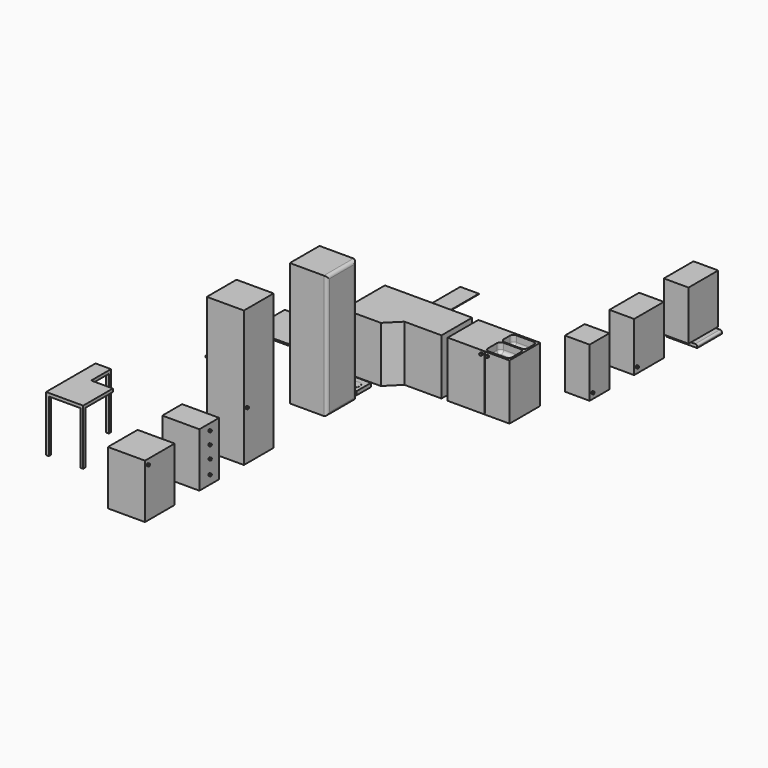
from build123d import *

# Parameters (mm, degrees)
F1_W           = 600
F1_H           = 600
F2_DEPTH       = 2000
F1_W_2         = 520
F1_H_2         = 290
F1_R           = 100
F1_R_2         = 80
F3_DEPTH       = 60
F4_DEPTH       = 900
F1_W_3         = 1000
F1_H_3         = 620
F5_DEPTH       = 900
F7_DEPTH       = 150
F8_R           = 50
F9_T           = 15
F10_DEPTH      = 61
F1_H_4         = 400
F11_DEPTH      = 875
F1_W_4         = 400
F1_H_5         = 50
F1_H_6         = 500
F12_DEPTH      = 800
F1_W_5         = 100
F13_DEPTH      = 50
F14_R          = 30
F15_DEPTH      = 800
F1_W_6         = 620
F1_H_7         = 700
F16_DEPTH      = 25
F17_R          = 20
F18_DEPTH      = 25
F19_DEPTH      = 2200
F20_R          = 20
F21_DEPTH      = 25
F22_R          = 50
F23_W          = 584
F23_H          = 870
F23_R          = 20
F23_W_2        = 385
F24_DEPTH      = 12
F25_DEPTH      = 25
F25_DEPTH_BACK = 12
F1_W_7         = 300
F1_H_8         = 900
F26_DEPTH      = 9
F1_W_8         = 45
F1_H_9         = 45
F27_DEPTH      = 50
F28_DEPTH      = 900


# Not quite as in the source:
# - a shell that OpenCascade refuses in one call is made with other operations: the cavity is built on its own and cut out


with BuildPart() as f2:
    # F1 (on Top) → F2 (new body)
    with BuildSketch(Plane.XY):
        with Locations((301, -1623.132034356)):
            Rectangle(F1_W, F1_H)
    extrude(amount=F2_DEPTH)

    # F22
    f22_edges = [f2.edges().sort_by_distance(p)[0] for p in [
        (601, -1923.132034, 1000),
        (601, -1323.132034, 1000),
        (601, -1623.132034, 2000),
        (601, -1623.132034, 0),
    ]]
    fillet(f22_edges, radius=F22_R)


with BuildPart() as f3:
    # F1 (on Top) → F3 (new body)
    with BuildSketch(Plane.XY):
        with Locations((261, -1078.132034356)):
            Rectangle(F1_W_2, F1_H_2)
        with Locations((181, -1073.132034356)):
            Circle(F1_R, mode=Mode.SUBTRACT)
        with Locations((391, -1093.132034356)):
            Circle(F1_R_2, mode=Mode.SUBTRACT)
    extrude(amount=F3_DEPTH)

    # F1 (on Top) → F10 (join)
    with BuildSketch(Plane.XY):
        with Locations((181, -1073.132034356)):
            Circle(F1_R)
        with Locations((391, -1093.132034356)):
            Circle(F1_R_2)
    extrude(amount=F10_DEPTH)


with BuildPart() as f4:
    # F1 (on Top) → F4 (new body)
    with BuildSketch(Plane.XY):
        Polygon((1, -833.132034356), (601, -833.132034356), (813.132034356, -621), (1413.132034356, -621), (1413.132034356, -1), (1, -1), align=None)
    extrude(amount=F4_DEPTH)


with BuildPart() as f5:
    # F1 (on Top) → F5 (new body)
    with BuildSketch(Plane.XY):
        with Locations((2013.132034356, -311)):
            Rectangle(F1_W_3, F1_H_3)
    extrude(amount=F5_DEPTH)

    # F6 (on face) → F7 (cut)
    with BuildSketch(Plane.XY.offset(900)):
        with BuildLine():
            Line((2423.132034356, -291), (2153.132034356, -291))
            ThreePointArc((2153.132034356, -291), (2110.7056274848, -308.5735931288), (2093.132034356, -351))
            Line((2093.132034356, -351), (2093.132034356, -531))
            ThreePointArc((2093.132034356, -531), (2110.7056274848, -573.4264068712), (2153.132034356, -591))
            Line((2153.132034356, -591), (2423.132034356, -591))
            ThreePointArc((2423.132034356, -591), (2465.5584412272, -573.4264068712), (2483.132034356, -531))
            Line((2483.132034356, -531), (2483.132034356, -351))
            ThreePointArc((2483.132034356, -351), (2465.5584412272, -308.5735931288), (2423.132034356, -291))
        make_face()
        with BuildLine():
            ThreePointArc((2093.132034356, -211), (2110.7056274848, -253.4264068712), (2153.132034356, -271))
            Line((2153.132034356, -271), (2423.132034356, -271))
            ThreePointArc((2423.132034356, -271), (2465.5584412272, -253.4264068712), (2483.132034356, -211))
            Line((2483.132034356, -211), (2483.132034356, -91))
            ThreePointArc((2483.132034356, -91), (2465.5584412272, -48.5735931288), (2423.132034356, -31))
            Line((2423.132034356, -31), (2153.132034356, -31))
            ThreePointArc((2153.132034356, -31), (2110.7056274848, -48.5735931288), (2093.132034356, -91))
            Line((2093.132034356, -91), (2093.132034356, -211))
        make_face()
    extrude(amount=-F7_DEPTH, mode=Mode.SUBTRACT)

    # F8
    f8_edges = [f5.edges().sort_by_distance(p)[0] for p in [
        (2288.132034, -291, 750),
        (2288.132034, -31, 750),
    ]]
    fillet(f8_edges, radius=F8_R)

    # F9: shell of thickness 15, made by hand


with BuildPart() as f9_core1:
    # F9_t2: copy of F5
    add(f5.part)

    # the walls: a layer under each face that stays
    f9_faces = [f9_core1.faces().sort_by_distance(p)[0] for p in [
        (2465.5584412272, -308.5735931288, 850),
        (2483.132034356, -441, 850),
        (2455.2031021678, -318.9289321881, 764.6446609407),
        (2013.132034356, -311, 900),
        (2288.132034356, -291, 850),
        (2465.5584412272, -573.4264068712, 850),
        (2468.4873734153, -441, 764.6446609407),
        (2288.132034356, -441, 750),
        (2288.132034356, -305.6446609407, 764.6446609407),
        (1513.132034356, -311, 450),
        (2513.132034356, -311, 450),
        (2013.132034356, -1, 450),
        (2110.7056274848, -308.5735931288, 850),
        (2093.132034356, -441, 850),
        (2110.7056274848, -573.4264068712, 850),
        (2288.132034356, -591, 850),
        (2110.7056274848, -48.5735931288, 850),
        (2093.132034356, -151, 850),
        (2110.7056274848, -253.4264068712, 850),
        (2288.132034356, -271, 850),
        (2465.5584412272, -253.4264068712, 850),
        (2483.132034356, -151, 850),
        (2465.5584412272, -48.5735931288, 850),
        (2288.132034356, -31, 850),
        (2455.2031021678, -563.0710678119, 764.6446609407),
        (2121.0609665441, -318.9289321881, 764.6446609407),
        (2107.7766952966, -441, 764.6446609407),
        (2121.0609665441, -563.0710678119, 764.6446609407),
        (2288.132034356, -576.3553390593, 764.6446609407),
        (2013.132034356, -311, 0),
        (2121.0609665441, -58.9289321881, 764.6446609407),
        (2107.7766952966, -151, 764.6446609407),
        (2121.0609665441, -243.0710678119, 764.6446609407),
        (2288.132034356, -256.3553390593, 764.6446609407),
        (2455.2031021678, -243.0710678119, 764.6446609407),
        (2468.4873734153, -151, 764.6446609407),
        (2455.2031021678, -58.9289321881, 764.6446609407),
        (2288.132034356, -45.6446609407, 764.6446609407),
        (2288.132034356, -151, 750),
    ]]
    thicken(f9_faces, amount=-F9_T, mode=Mode.SUBTRACT)


with BuildPart() as f5_1:
    add(f5.part)

    # what is left inside the walls is the cavity
    f9_cavity = [f9_core1.part.solids().sort_by_distance(p)[0] for p in [
        (2013.132034, -620.85, 595),
    ]]
    add(f9_cavity, mode=Mode.SUBTRACT)

    # F23 (on face) → F24 (join)
    with BuildSketch(Plane.XZ.offset(621)):
        with Locations((1820.132034356, 450)):
            Rectangle(F23_W, F23_H)
        with Locations((2063.132034356, 850)):
            Circle(F23_R, mode=Mode.SUBTRACT)
        with Locations((2305.632034356, 450)):
            Rectangle(F23_W_2, F23_H)
        with Locations((2163.132034356, 850)):
            Circle(F23_R, mode=Mode.SUBTRACT)
    extrude(amount=-F24_DEPTH)

    # F23 (on face) → F25 (join, two sides)
    with BuildSketch(Plane.XZ.offset(621)) as f25_sk:
        with Locations((2063.132034356, 850)):
            Circle(F23_R)
        with Locations((2163.132034356, 850)):
            Circle(F23_R)
    extrude(amount=F25_DEPTH)
    extrude(f25_sk.sketch, amount=-F25_DEPTH_BACK)


with BuildPart() as f11:
    # F1 (on Top) → F11 (new body)
    with BuildSketch(Plane.XY):
        with Locations((300, -4300)):
            Rectangle(F1_W, F1_H_4)
    extrude(amount=F11_DEPTH)

    # F20 (on face) → F21, piece 2 (join)
    with BuildSketch(Plane.YZ.offset(600)):
        with Locations((-4300, 150)):
            Circle(F20_R)
        with Locations((-4300, 375)):
            Circle(F20_R)
        with Locations((-4300, 575)):
            Circle(F20_R)
        with Locations((-4300, 775)):
            Circle(F20_R)
    extrude(amount=F21_DEPTH)


with BuildPart() as f11b:
    # F1 (on Top) → F11, piece 2 (new body)
    with BuildSketch(Plane.XY):
        with Locations((300, -5300)):
            Rectangle(F1_W, F1_H)
    extrude(amount=F11_DEPTH)

    # F20 (on face) → F21, piece 3 (join)
    with BuildSketch(Plane.YZ.offset(600)):
        with Locations((-5550, 800)):
            Circle(F20_R)
    extrude(amount=F21_DEPTH)


with BuildPart() as f12:
    # F1 (on Top) → F12 (new body)
    with BuildSketch(Plane.XY):
        with Locations((2713.132034356, 3074)):
            Rectangle(F1_W_4, F1_H_5)
        with Locations((2713.132034356, 2799)):
            Rectangle(F1_W_4, F1_H_6)
        with Locations((2713.132034356, 2524)):
            Rectangle(F1_W_4, F1_H_5)
    extrude(amount=F12_DEPTH)

    # F1 (on Top) → F13 (join)
    with BuildSketch(Plane.XY):
        with Locations((2963.132034356, 2799)):
            Rectangle(F1_W_5, F1_H_6)
        with Locations((2713.132034356, 2799)):
            Rectangle(F1_W_4, F1_H_6)
    extrude(amount=-F13_DEPTH)

    # F14
    f14_edges = [f12.edges().sort_by_distance(p)[0] for p in [
        (3013.132034, 2799, 0),
    ]]
    fillet(f14_edges, radius=F14_R)


with BuildPart() as f15:
    # F1 (on Top) → F15 (new body)
    with BuildSketch(Plane.XY):
        with Locations((2713.132034356, 699)):
            Rectangle(F1_W_4, F1_H_4)
    extrude(amount=F15_DEPTH)

    # F17 (on face) → F18 (join)
    with BuildSketch(Plane.YZ.offset(2913.132034356)):
        with Locations((549, 100)):
            Circle(F17_R)
    extrude(amount=F18_DEPTH)


with BuildPart() as f15b:
    # F1 (on Top) → F15, piece 2 (new body)
    with BuildSketch(Plane.XY):
        with Locations((2713.132034356, 1699)):
            Rectangle(F1_W_4, F1_H)
    extrude(amount=F15_DEPTH)

    # F17 (on face) → F18, piece 2 (join)
    with BuildSketch(Plane.YZ.offset(2913.132034356)):
        with Locations((1449, 100)):
            Circle(F17_R)
    extrude(amount=F18_DEPTH)


with BuildPart() as f16:
    # F1 (on Top) → F16 (new body)
    with BuildSketch(Plane.XY):
        with Locations((-1310, -350)):
            Rectangle(F1_W_6, F1_H_7)
    extrude(amount=F16_DEPTH)


with BuildPart() as f16b:
    # F1 (on Top) → F16, piece 2 (new body)
    with BuildSketch(Plane.XY):
        with Locations((-1310, -1400)):
            Rectangle(F1_W_6, F1_H_4)
    extrude(amount=F16_DEPTH)


with BuildPart() as f19:
    # F1 (on Top) → F19 (new body)
    with BuildSketch(Plane.XY):
        with Locations((300, -3300)):
            Rectangle(F1_W, F1_H)
    extrude(amount=F19_DEPTH)

    # F20 (on face) → F21 (join)
    with BuildSketch(Plane.YZ.offset(600)):
        with Locations((-3550, 800)):
            Circle(F20_R)
    extrude(amount=F21_DEPTH)


with BuildPart() as f26:
    # F1 (on Top) → F26 (new body)
    with BuildSketch(Plane.XY):
        with Locations((-150, 1450)):
            Rectangle(F1_W_7, F1_H_8)
    extrude(amount=F26_DEPTH)


with BuildPart() as f27:
    # F1 (on Top) → F27 (new body)
    with BuildSketch(Plane.XY):
        Polygon((-2350, -3000), (-2350, -2645), (-2395, -2645), (-2395, -2600), (-2600, -2600), (-2600, -3555), (-2555, -3555), (-2555, -3600), (-2045, -3600), (-2045, -3555), (-2000, -3555), (-2000, -3000), align=None)
        with Locations((-2372.5, -2622.5)):
            Rectangle(F1_W_8, F1_H_9)
        with Locations((-2577.5, -3577.5)):
            Rectangle(F1_W_8, F1_H_9)
        with Locations((-2022.5, -3577.5)):
            Rectangle(F1_W_8, F1_H_9)
    extrude(amount=-F27_DEPTH)

    # F1 (on Top) → F28 (join)
    with BuildSketch(Plane.XY):
        with Locations((-2577.5, -3577.5)):
            Rectangle(F1_W_8, F1_H_9)
        with Locations((-2022.5, -3577.5)):
            Rectangle(F1_W_8, F1_H_9)
        with Locations((-2372.5, -2622.5)):
            Rectangle(F1_W_8, F1_H_9)
    extrude(amount=-F28_DEPTH)


solid = Compound([f2.part, f3.part, f4.part, f5_1.part, f11.part, f11b.part, f12.part, f15.part, f15b.part, f16.part, f16b.part, f19.part, f26.part, f27.part])
